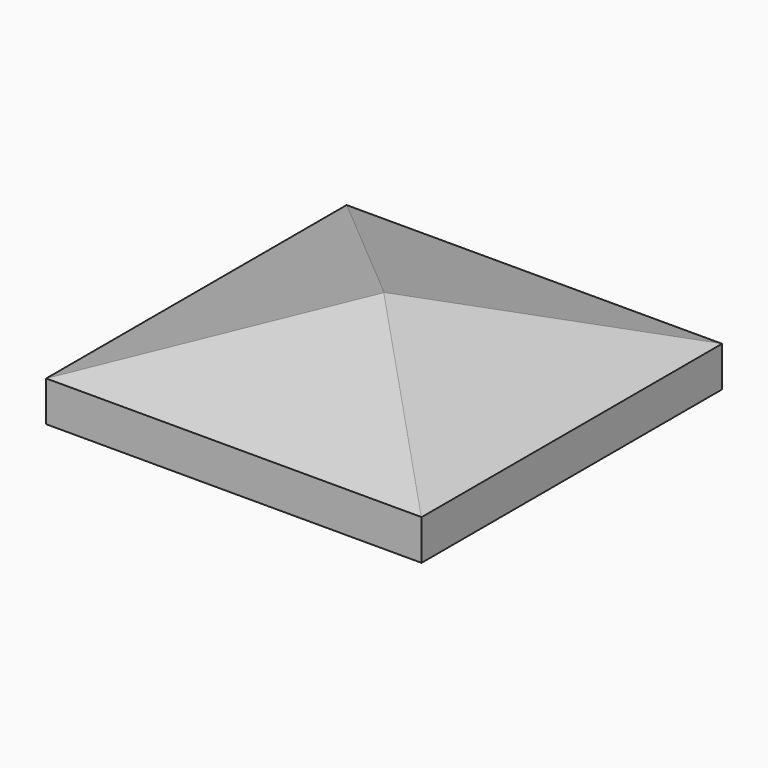
from build123d import *

# Parameters (mm, degrees)
F0_W     = 177.8
F0_H     = 177.8
F1_DEPTH = 47.625
F4_DEPTH = 177.801
F5_DEPTH = 177.801


# Not quite as in the source:
# - ends of sketch curves that miss each other by under 0.0002 mm in the source are joined


with BuildPart() as f1:
    # F0 (on Top) → F1 (new body)
    with BuildSketch(Plane.XY):
        with Locations((-88.9, 88.9)):
            Rectangle(F0_W, F0_H)
    extrude(amount=F1_DEPTH)

    # F3 (on face) → F4 (cut, through all)
    with BuildSketch(Plane(origin=(-177.8, 0, 0), x_dir=(0, -1, 0), z_dir=(-1, 0, 0))):
        Polygon((-177.8, 47.625), (-177.8, 19.0884657204), (-89.0196708441, 47.625), align=None)
        Polygon((-88.7803285837, 47.625), (2.861e-07, 19.0884657204), (0, 47.625), align=None)
    extrude(amount=-F4_DEPTH, mode=Mode.SUBTRACT)

    # F2 (on face) → F5 (cut, through all)
    with BuildSketch(Plane.XZ):
        Polygon((-177.8, 19.05), (-88.9, 47.625), (-177.8, 47.625), align=None)
        Polygon((-88.9, 47.625), (0, 19.05), (0, 47.625), align=None)
    extrude(amount=-F5_DEPTH, mode=Mode.SUBTRACT)


solid = f1.part
